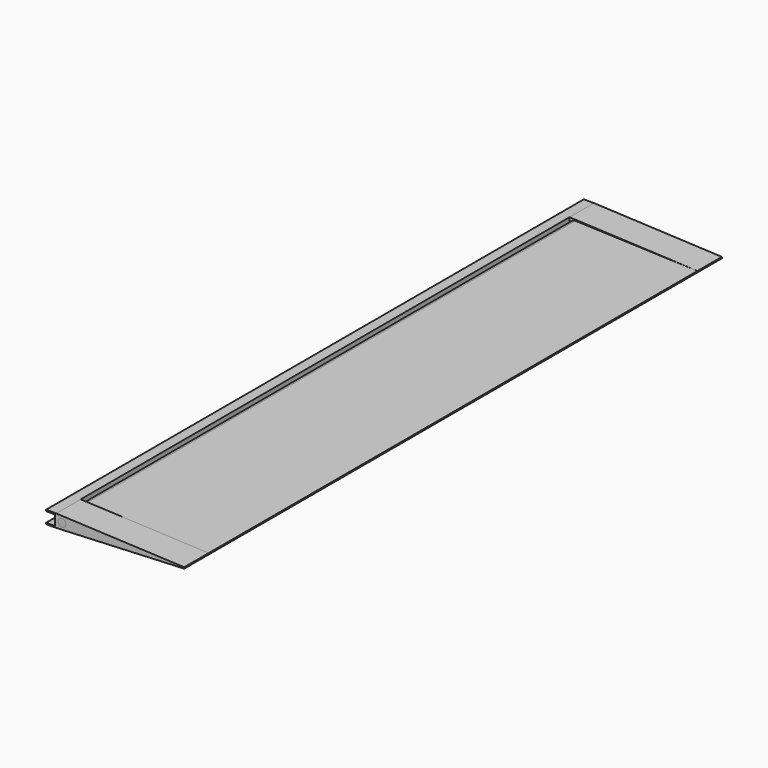
from build123d import *

# Parameters (mm, degrees)
F0_R     = 9.525
F1_DEPTH = 762
F2_DEPTH = 838.2
F4_DEPTH = 838.2
F5_R     = 9.525
F6_DEPTH = 76.2


# Not quite as in the source:
# - a pattern or mirror of a feature is missing from the dataset's text; its kind, count and spacing are read off the source's solid


with BuildPart() as f1:
    # F0 (on Front) → F1 (new body, symmetric)
    with BuildSketch(Plane.XZ):
        with BuildLine():
            Line((304.8, 1.5875), (0.4630648172, 12.6915551047))
            ThreePointArc((0.4630648172, 12.6915551047), (-12.7, 0), (0.4630648172, -12.6915551047))
            Line((0.4630648172, -12.6915551047), (304.8, -1.5875))
            Line((304.8, -1.5875), (304.8, 1.5875))
        make_face()
        Circle(F0_R, mode=Mode.SUBTRACT)
        Circle(F0_R)
    extrude(amount=F1_DEPTH, both=True)

    # F0 (on Front) → F2 (join, symmetric)
    with BuildSketch(Plane.XZ):
        Circle(F0_R)
    extrude(amount=F2_DEPTH, both=True)


with BuildPart() as f4:
    # F3 (on Front) → F4 (new body, symmetric)
    with BuildSketch(Plane.XZ):
        Polygon((-14.2875, -15.875), (-14.2875, 15.875), (-39.6875, 15.875), (-39.6875, 12.7), (-17.4625, 12.7), (-17.4625, -12.7), (-39.6875, -12.7), (-39.6875, -15.875), align=None)
    extrude(amount=F4_DEPTH, both=True)

    # F5 (on face) → F6 (join)
    with BuildSketch(Plane.XZ.offset(762)):
        Polygon((304.8, -1.5875), (304.8, 1.5875), (-14.2875, 15.875), (-14.2875, -15.875), align=None)
        Circle(F5_R, mode=Mode.SUBTRACT)
    f6 = extrude(amount=F6_DEPTH)

    # F6_copies: F6 across plane
    add(f6.mirror(Plane.ZX))


solid = Compound([f1.part, f4.part])
